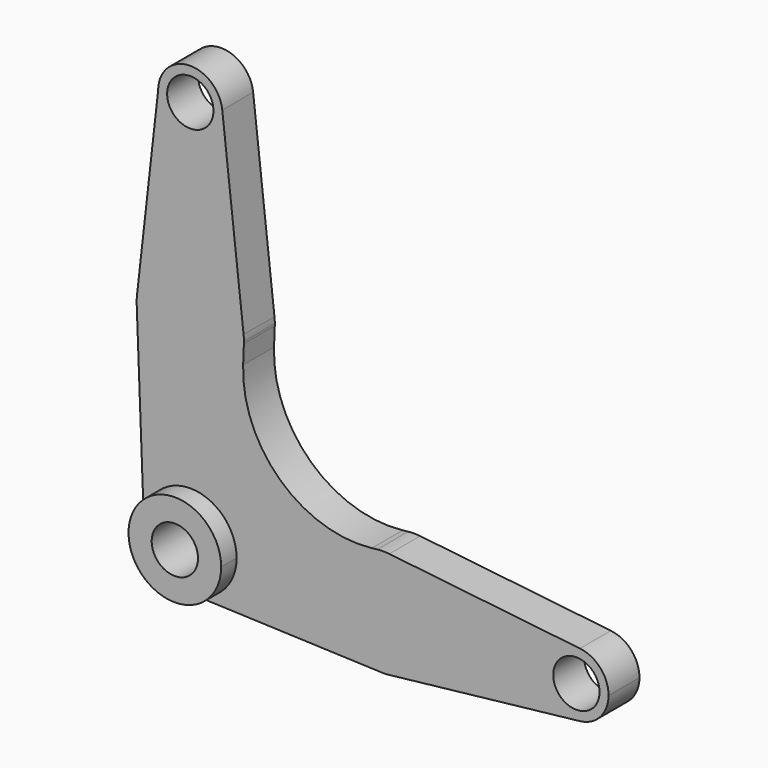
from build123d import *

# Parameters (mm, degrees)
F0_R     = 3.81
F1_DEPTH = 6.35
F2_R     = 3.81
F3_DEPTH = 3.175


# Not quite as in the source:
# - a feature names something its author has since deleted; it is built from what else it names


with BuildPart() as f1:
    # F0 (on Front) → F1 (new body)
    with BuildSketch(Plane.XZ):
        with BuildLine():
            ThreePointArc((64.087961787, 5.2589050049), (58.2083291, 0), (64.087961787, -5.2589050049))
            ThreePointArc((64.087961787, -5.2589050049), (67.4441780635, -3.5277812174), (68.7916709, 0))
            ThreePointArc((68.7916709, 0), (67.4441780635, 3.5277812174), (64.087961787, 5.2589050049))
        make_face()
        with Locations((63.5, 0)):
            Circle(F0_R, mode=Mode.SUBTRACT)
        with BuildLine():
            ThreePointArc((5.2589006137, 64.087962963), (5.2834688034, 63.794437625), (5.2916666667, 63.5))
            ThreePointArc((5.2916666667, 63.5), (0, 58.2083333333), (-5.2916666667, 63.5))
            Line((-5.2916666667, 63.5), (-8.7637923714, 32.7392136171))
            ThreePointArc((-8.7637923714, 32.7392136171), (0.0046668449, 40.5694432097), (8.7648343562, 32.7299382716))
            Line((8.7648343562, 32.7299382716), (5.2589006137, 64.087962963))
        make_face()
        with BuildLine():
            ThreePointArc((-5.2916666667, 63.5), (0, 58.2083333333), (5.2916666667, 63.5))
            ThreePointArc((5.2916666667, 63.5), (5.2834688034, 63.794437625), (5.2589006137, 64.087962963))
            ThreePointArc((5.2589006137, 64.087962963), (-0.294437625, 68.7834688034), (-5.2916666667, 63.5))
        make_face()
        with Locations((0, 63.5)):
            Circle(F0_R, mode=Mode.SUBTRACT)
        with BuildLine():
            ThreePointArc((8.8131488161, 31.4168209877), (0, 22.9305555556), (-8.8131488161, 31.4168209877))
            Line((-8.8131488161, 31.4168209877), (-7.6145605771, -0.2878666667))
            ThreePointArc((-7.6145605771, -0.2878666667), (-0.1439590264, 7.6186400229), (7.62, 0))
            ThreePointArc((7.62, 0), (5.3881536726, -5.3881536726), (0, -7.62))
            Line((0, -7.62), (31.4152979668, -8.8130854583))
            ThreePointArc((31.4152979668, -8.8130854583), (22.9364968819, -0.3235174392), (30.7700650994, 8.7648290535))
            Line((30.7700650994, 8.7648290535), (29.8488925204, 8.6618391202))
            ThreePointArc((29.8488925204, 8.6618391202), (14.7662444168, 13.637318243), (8.6958303376, 28.313548659))
            Line((8.6958303376, 28.313548659), (8.8131488161, 31.4168209877))
        make_face()
        with BuildLine():
            ThreePointArc((30.7700650994, 8.7648290535), (22.9364968819, -0.3235174392), (31.4152979668, -8.8130854583))
            ThreePointArc((31.4152979668, -8.8130854583), (32.0735174392, -8.8135031181), (32.7299349006, -8.7648290535))
            ThreePointArc((32.7299349006, -8.7648290535), (38.3236206398, -5.8796268956), (40.5694388, 0))
            ThreePointArc((40.5694388, 0), (38.3236206398, 5.8796268956), (32.7299349006, 8.7648290535))
            ThreePointArc((32.7299349006, 8.7648290535), (31.75, 8.8194388), (30.7700650994, 8.7648290535))
        make_face()
        with BuildLine():
            ThreePointArc((40.5694388, 0), (38.3236206398, -5.8796268956), (32.7299349006, -8.7648290535))
            Line((32.7299349006, -8.7648290535), (64.087961787, -5.2589050049))
            ThreePointArc((64.087961787, -5.2589050049), (58.2083291, 0), (64.087961787, 5.2589050049))
            Line((64.087961787, 5.2589050049), (32.7299349006, 8.7648290535))
            ThreePointArc((32.7299349006, 8.7648290535), (38.3236206398, 5.8796268956), (40.5694388, 0))
        make_face()
        with BuildLine():
            ThreePointArc((7.62, 0), (-0.1439590264, 7.6186400229), (-7.6145605771, -0.2878666667))
            ThreePointArc((-7.6145605771, -0.2878666667), (-5.2853976199, -5.4889864274), (0, -7.62))
            ThreePointArc((0, -7.62), (5.3881536726, -5.3881536726), (7.62, 0))
        make_face()
        Circle(F0_R, mode=Mode.SUBTRACT)
        with BuildLine():
            ThreePointArc((8.8194444444, 31.75), (8.8057813389, 32.240729375), (8.7648343562, 32.7299382716))
            ThreePointArc((8.7648343562, 32.7299382716), (0.0046668449, 40.5694432097), (-8.7637923714, 32.7392136171))
            ThreePointArc((-8.7637923714, 32.7392136171), (-8.8133078888, 32.0789443195), (-8.8131488161, 31.4168209877))
            ThreePointArc((-8.8131488161, 31.4168209877), (0, 22.9305555556), (8.8131488161, 31.4168209877))
            ThreePointArc((8.8131488161, 31.4168209877), (8.8178703969, 31.5833807565), (8.8194444444, 31.75))
        make_face()
    extrude(amount=F1_DEPTH)

    # F2 (on face) → F3 (join)
    with BuildSketch(Plane.XZ.offset(6.35)):
        with BuildLine():
            ThreePointArc((0, -7.62), (5.3881536726, -5.3881536726), (7.62, 0))
            ThreePointArc((7.62, 0), (-0.1439590264, 7.6186400229), (-7.6145605771, -0.2878666667))
            ThreePointArc((-7.6145605771, -0.2878666667), (-5.2853976199, -5.4889864274), (0, -7.62))
        make_face()
        Circle(F2_R, mode=Mode.SUBTRACT)
    extrude(amount=F3_DEPTH)


solid = f1.part
